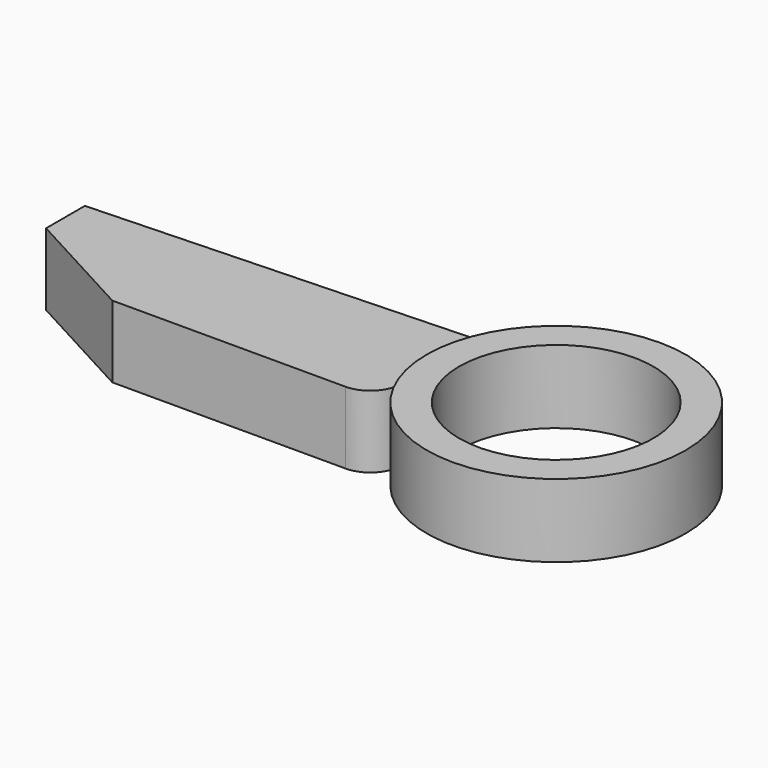
from build123d import *

# Parameters (mm, degrees)
F0_R        = 21.1613086429
F1_DEPTH    = 11.9615718722
F3_DEPTH    = 11.6841569543
F4_T1_DEPTH = 36.288056526
F6_DEPTH    = 0.0834609382
F10_D       = 31.75


# Not quite as in the source:
# - a fillet or chamfer that OpenCascade refuses, or shapes differently, is made with other operations: its cross-section is extruded or revolved along the edge and cut away or added
# - the program builds the solid bodies; features that only make, move or delete a surface that nothing else refers to are left out


with BuildPart() as f1:
    # F0 (on Top) → F1 (new body)
    with BuildSketch(Plane.XY):
        Circle(F0_R)
    extrude(amount=F1_DEPTH)

    # F2 (on Top) → F3 (join)
    with BuildSketch(Plane.XY):
        Polygon((-19.0119333565, -13.1104551256), (-19.0119333565, 7.5374748558), (-36.1838054091, 6.8717853914), (-59.2216673993, 5.9786933651), (-81.0971707106, 5.1306616515), (-81.0971707106, -2.7903839946), (-62.0231479406, -13.1104551256), align=None)
    extrude(amount=F3_DEPTH)

    # F4: fillet of radius 5.08 on 1 edges, made by hand

    # F4_s2 → F4_t1 (cut)
    with BuildSketch(Plane.XY.offset(-12.3019497859)):
        with BuildLine():
            ThreePointArc((-19.0119333565, -9.2923287462), (-20.8185454842, -12.0439771445), (-23.9327132709, -13.1104551256))
            Line((-23.9327132709, -13.1104551256), (-19.0119333565, -13.1104551256))
            Line((-19.0119333565, -13.1104551256), (-19.0119333565, -9.2923287462))
        make_face()
    extrude(amount=F4_T1_DEPTH, mode=Mode.SUBTRACT)

    # F5 (on face) → F6 (join)
    with BuildSketch(Plane.XY.offset(11.6841569543)):
        with BuildLine():
            ThreePointArc((-19.0119333565, -9.2923287462), (-21.1389513114, -0.9724818434), (-19.7847977051, 7.5075137862))
            Line((-19.7847977051, 7.5075137862), (-81.0971707106, 5.1306616515))
            Line((-81.0971707106, 5.1306616515), (-81.0971707106, -2.7903839946))
            Line((-81.0971707106, -2.7903839946), (-62.0231479406, -13.1104551256))
            Line((-62.0231479406, -13.1104551256), (-23.9327132709, -13.1104551256))
            ThreePointArc((-23.9327132709, -13.1104551256), (-20.8185454842, -12.0439771445), (-19.0119333565, -9.2923287462))
        make_face()
    extrude(amount=F6_DEPTH)

    # F10 (through all)
    with Locations(Plane.XY.offset(11.9615718722)):
        with Locations((0, 0)):
            Hole(F10_D / 2)


solid = f1.part
